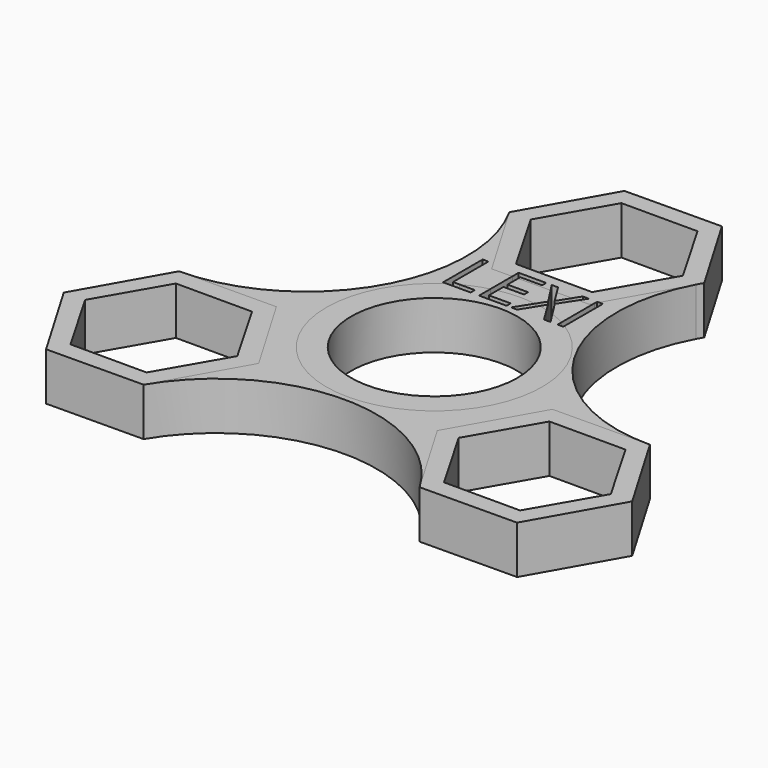
from build123d import *

# Parameters (mm, degrees)
F1_R         = 14.2875
F2_DEPTH     = 6.35
F0_R         = 14.2875
F0_R_2       = 11.0236
F3_TEXT_SIZE = 9.1819106368
F4_DEPTH     = 25.4


# Not quite as in the source:
# - a feature names something its author has since deleted; it is built from what else it names
# - Text() gives the source's letters only with a copy of the font that has no kerning and outlines rounded to 1/6400 em; it was checked with that copy


with BuildPart() as f2:
    # F1 (on Top) → F2 (new body)
    with BuildSketch(Plane.XY):
        with BuildLine():
            Line((11.9154897652, -14.3917610701), (18.2407901039, -3.2274973703))
            Line((18.2407901039, -3.2274973703), (31.0719762518, -3.1232363002))
            ThreePointArc((31.0719762518, -3.1232363002), (12.8883108864, 7.0476864321), (12.3762552757, 27.8763002697))
            Line((12.3762552757, 27.8763002697), (6.5058858093, 17.5149973703))
            Line((6.5058858093, 17.5149973703), (-6.3253003386, 17.4107363002))
            Line((-6.3253003386, 17.4107363002), (-12.8311861479, 28.4707389299))
            ThreePointArc((-12.8311861479, 28.4707389299), (-13.0069185167, 7.3709719586), (-31.2525617224, -3.2274973703))
            Line((-31.2525617224, -3.2274973703), (-18.4213755745, -3.1232363002))
            Line((-18.4213755745, -3.1232363002), (-11.9154897652, -14.1832389299))
            Line((-11.9154897652, -14.1832389299), (-18.2407901039, -25.3475026297))
            ThreePointArc((-18.2407901039, -25.3475026297), (0.1200102916, -14.9498078397), (18.4213755745, -25.4517636998))
            Line((18.4213755745, -25.4517636998), (11.9154897652, -14.3917610701))
        make_face()
        Circle(F1_R, mode=Mode.SUBTRACT)
    extrude(amount=F2_DEPTH)


with BuildPart() as f2b:
    # F0 (on Top) → F2, piece 2 (new body)
    with BuildSketch(Plane.XY):
        Circle(F0_R)
        Circle(F0_R_2, mode=Mode.SUBTRACT)
    extrude(amount=F2_DEPTH)


with BuildPart() as f2c:
    # F0 (on Top) → F2, piece 3 (new body)
    with BuildSketch(Plane.XY):
        Polygon((12.8311861479, 28.6792610701), (6.3253003386, 39.7392636998), (-6.5058858093, 39.6350026297), (-12.8311861479, 28.4707389299), (-6.3253003386, 17.4107363002), (6.5058858093, 17.5149973703), align=None)
        Polygon((-10.0819790757, 28.575), (-5.0409895379, 37.30625), (5.0409895379, 37.30625), (10.0819790757, 28.575), (5.0409895379, 19.84375), (-5.0409895379, 19.84375), align=None, mode=Mode.SUBTRACT)
    extrude(amount=F2_DEPTH)


with BuildPart() as f2d:
    # F0 (on Top) → F2, piece 4 (new body)
    with BuildSketch(Plane.XY):
        Polygon((-31.0719762518, -25.4517636998), (-18.2407901039, -25.3475026297), (-11.9154897652, -14.1832389299), (-18.4213755745, -3.1232363002), (-31.2525617224, -3.2274973703), (-37.5778620611, -14.3917610701), align=None)
        Polygon((-14.6646968374, -14.2875), (-19.7056863753, -23.01875), (-29.787665451, -23.01875), (-34.8286549889, -14.2875), (-29.787665451, -5.55625), (-19.7056863753, -5.55625), align=None, mode=Mode.SUBTRACT)
    extrude(amount=F2_DEPTH)


with BuildPart() as f2e:
    # F0 (on Top) → F2, piece 5 (new body)
    with BuildSketch(Plane.XY):
        Polygon((37.5778620611, -14.1832389299), (31.0719762518, -3.1232363002), (18.2407901039, -3.2274973703), (11.9154897652, -14.3917610701), (18.4213755745, -25.4517636998), (31.2525617224, -25.3475026297), align=None)
        Polygon((19.7056863753, -5.55625), (29.787665451, -5.55625), (34.8286549889, -14.2875), (29.787665451, -23.01875), (19.7056863753, -23.01875), (14.6646968374, -14.2875), align=None, mode=Mode.SUBTRACT)
    extrude(amount=F2_DEPTH)


with BuildPart() as f4_tool:
    # F3 (on face) → F4 (new body)
    with BuildSketch(Plane.XY.offset(6.35)):
        with Locations((-9.2717003121, 11.9221359491)):
            Text('LEXI', F3_TEXT_SIZE, font='Open Sans', text_align=(TextAlign.LEFT, TextAlign.BOTTOM))
    extrude(amount=-F4_DEPTH)


with BuildPart() as f2_1:
    add(f2.part)

    # F4: cut by f4_tool
    add(f4_tool.part, mode=Mode.SUBTRACT)


with BuildPart() as f2b_1:
    add(f2b.part)

    # F4: cut by f4_tool
    add(f4_tool.part, mode=Mode.SUBTRACT)


with BuildPart() as f2c_1:
    add(f2c.part)

    # F4: cut by f4_tool
    add(f4_tool.part, mode=Mode.SUBTRACT)


solid = Compound([f2d.part, f2e.part, f2_1.part, f2b_1.part, f2c_1.part])
